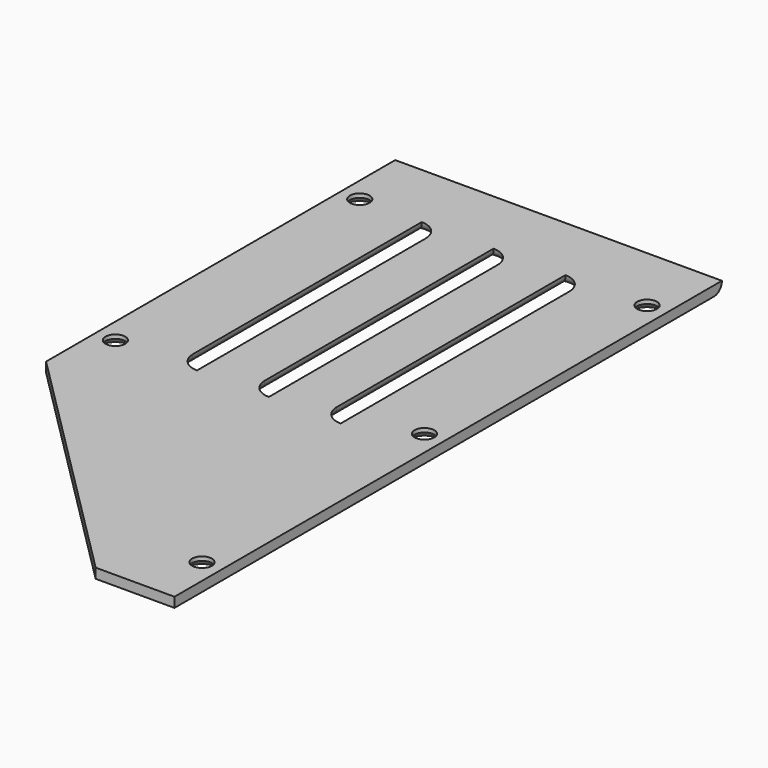
from build123d import *

# Parameters (mm, degrees)
F0_R     = 2.5
F1_DEPTH = 1.25
F2_R     = 2.49999
F3_SIZE  = 1.5


# Not quite as in the source:
# - a fillet or chamfer is up to 0.001 mm smaller than in the source, because OpenCascade refuses the exact size


with BuildPart() as f1:
    # F0 (on Top) → F1 (new body, symmetric)
    with BuildSketch(Plane.XY):
        Polygon((41.4535664022, 86.8200212717), (-41.4534695446, 86.8200212717), (-41.4534695446, -23.9119753242), (21.4531961828, -86.8199840188), (41.4535664022, -86.8199840188), align=None)
        with Locations((-36.4534695446, -8.1799787283)):
            Circle(F0_R, mode=Mode.SUBTRACT)
        with Locations((36.4535664022, -71.8299787283)):
            Circle(F0_R, mode=Mode.SUBTRACT)
        with Locations((36.4535664022, -1.2799787283)):
            Circle(F0_R, mode=Mode.SUBTRACT)
        with BuildLine():
            Line((-20.7270524408, -3.1985588427), (-20.7270524408, 69.3289190531))
            ThreePointArc((-20.7270524408, 69.3289190531), (-17.1909272701, 67.8581418384), (-15.7270524408, 64.3191536607))
            Line((-15.7270524408, 64.3191536607), (-15.7270524408, -8.1787062808))
            ThreePointArc((-15.7270524408, -8.1787062808), (-19.2613774966, -6.7270807891), (-20.7270524408, -3.1985588427))
        make_face(mode=Mode.SUBTRACT)
        with BuildLine():
            Line((-2.5020524408, -3.1985588427), (-2.5020524408, 69.3289190531))
            ThreePointArc((-2.5020524408, 69.3289190531), (1.0340727299, 67.8581418384), (2.4979475592, 64.3191536607))
            Line((2.4979475592, 64.3191536607), (2.4979475592, -8.1787062808))
            ThreePointArc((2.4979475592, -8.1787062808), (-1.0363774966, -6.7270807891), (-2.5020524408, -3.1985588427))
        make_face(mode=Mode.SUBTRACT)
        with Locations((-36.4534695446, 69.3200212717)):
            Circle(F0_R, mode=Mode.SUBTRACT)
        with BuildLine():
            Line((15.7229475592, -3.1985588427), (15.7229475592, 69.3289190531))
            ThreePointArc((15.7229475592, 69.3289190531), (19.2590727299, 67.8581418384), (20.7229475592, 64.3191536607))
            Line((20.7229475592, 64.3191536607), (20.7229475592, -8.1787062808))
            ThreePointArc((20.7229475592, -8.1787062808), (17.1886225034, -6.7270807891), (15.7229475592, -3.1985588427))
        make_face(mode=Mode.SUBTRACT)
        with Locations((36.4535664022, 69.3200212717)):
            Circle(F0_R, mode=Mode.SUBTRACT)
    extrude(amount=F1_DEPTH, both=True)

    # F2 (radius 2.5 in the source; OpenCascade refuses exactly that, so slightly less here)
    f2_edges = [f1.edges().sort_by_distance(p)[0] for p in [
        (4.8e-05, 86.820021, -1.25),
        (-2.502052, 33.06518, -1.25),
        (2.497948, 28.070224, -1.25),
        (-20.727052, 33.06518, -1.25),
        (-15.727052, 28.070224, -1.25),
        (15.722948, 33.06518, -1.25),
        (20.722948, 28.070224, -1.25),
    ]]
    fillet(f2_edges, radius=F2_R)

    # F3
    f3_edges = [f1.edges().sort_by_distance(p)[0] for p in [
        (-38.95347, 69.320021, -1.25),
        (33.953566, 69.320021, -1.25),
        (33.953566, -1.279979, -1.25),
        (-38.95347, -8.179979, -1.25),
        (33.953566, -71.829979, -1.25),
    ]]
    chamfer(f3_edges, length=F3_SIZE)


solid = f1.part
